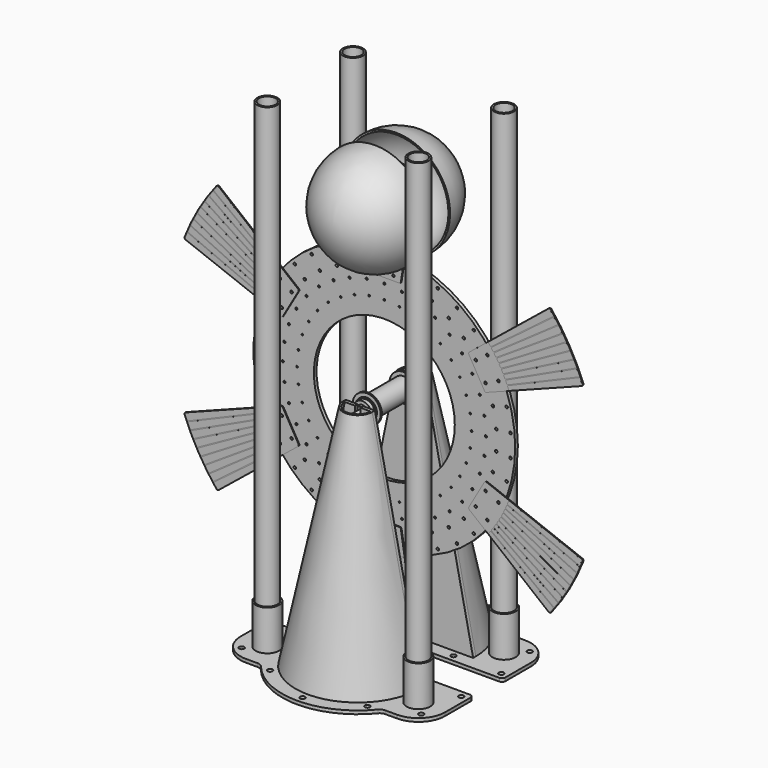
from build123d import *

# Parameters (mm, degrees)
F0_R      = 247.65
F0_R_2    = 2.38125
F0_R_3    = 1.9939
F0_R_4    = 1.5875
F0_R_5    = 133.35
F1_DEPTH  = 3.175
F2_R      = 2.38125
F3_DEPTH  = 1.5875
F5_DEPTH  = 0.0254
F8_COUNT  = 6
F13_DEPTH = 6.35
F14_DEPTH = 6.35
F15_ANGLE = 180
F16_R     = 4.7625
F16_R_2   = 22.225
F16_R_3   = 19.05
F16_R_4   = 15.875
F17_DEPTH = 6.35
F18_DEPTH = 76.2
F19_DEPTH = 908.05


with BuildPart() as f1:
    # F0 (on Front) → F1 (new body, symmetric)
    with BuildSketch(Plane.XZ):
        Circle(F0_R)
        with Locations((-137.4934414988, -196.3609844166)):
            Circle(F0_R_2, mode=Mode.SUBTRACT)
        with Locations((-196.3609844166, -137.4934414988)):
            Circle(F0_R_2, mode=Mode.SUBTRACT)
        with Locations((-169.5023342852, -169.5023342852)):
            Circle(F0_R_2, mode=Mode.SUBTRACT)
        with Locations((-150.4192900279, -150.4192900279)):
            Circle(F0_R_2, mode=Mode.SUBTRACT)
        with Locations((-101.3068800675, -217.2533054)):
            Circle(F0_R_2, mode=Mode.SUBTRACT)
        with Locations((-62.0421603491, -231.5444946343)):
            Circle(F0_R_2, mode=Mode.SUBTRACT)
        with Locations((-89.9014697288, -192.7943239974)):
            Circle(F0_R_2, mode=Mode.SUBTRACT)
        with Locations((-20.8923209834, -238.8003215663)):
            Circle(F0_R_2, mode=Mode.SUBTRACT)
        with Locations((-55.0572813694, -205.4765713973)):
            Circle(F0_R_2, mode=Mode.SUBTRACT)
        with Locations((-33.3715277272, -189.2593384922)):
            Circle(F0_R_3, mode=Mode.SUBTRACT)
        with Locations((-18.540205376, -211.9155171516)):
            Circle(F0_R_2, mode=Mode.SUBTRACT)
        with Locations((-122.0140474228, -174.2541186214)):
            Circle(F0_R_2, mode=Mode.SUBTRACT)
        with Locations((-96.0894844264, -166.4318690996)):
            Circle(F0_R_3, mode=Mode.SUBTRACT)
        with Locations((-65.7290784712, -180.5891589012)):
            Circle(F0_R_3, mode=Mode.SUBTRACT)
        with Locations((-123.5302600209, -147.217631174)):
            Circle(F0_R_3, mode=Mode.SUBTRACT)
        with Locations((-106.1242343592, -126.4739375589)):
            Circle(F0_R_4, mode=Mode.SUBTRACT)
        with Locations((-82.55, -142.9807941648)):
            Circle(F0_R_4, mode=Mode.SUBTRACT)
        with Locations((-56.4675256631, -155.1432516918)):
            Circle(F0_R_4, mode=Mode.SUBTRACT)
        with Locations((-28.6693141328, -162.5917600223)):
            Circle(F0_R_4, mode=Mode.SUBTRACT)
        with Locations((-217.2533054, -101.3068800675)):
            Circle(F0_R_2, mode=Mode.SUBTRACT)
        with Locations((-231.5444946343, -62.0421603491)):
            Circle(F0_R_2, mode=Mode.SUBTRACT)
        with Locations((-192.7943239974, -89.9014697288)):
            Circle(F0_R_2, mode=Mode.SUBTRACT)
        with Locations((-174.2541186214, -122.0140474228)):
            Circle(F0_R_2, mode=Mode.SUBTRACT)
        with Locations((-166.4318690996, -96.0894844264)):
            Circle(F0_R_3, mode=Mode.SUBTRACT)
        with Locations((-147.217631174, -123.5302600209)):
            Circle(F0_R_3, mode=Mode.SUBTRACT)
        with Locations((-126.4739375589, -106.1242343592)):
            Circle(F0_R_4, mode=Mode.SUBTRACT)
        with Locations((-180.5891589012, -65.7290784712)):
            Circle(F0_R_3, mode=Mode.SUBTRACT)
        with Locations((-142.9807941648, -82.55)):
            Circle(F0_R_4, mode=Mode.SUBTRACT)
        with Locations((-205.4765713973, -55.0572813694)):
            Circle(F0_R_2, mode=Mode.SUBTRACT)
        with Locations((-189.2593384922, -33.3715277272)):
            Circle(F0_R_3, mode=Mode.SUBTRACT)
        with Locations((-238.8003215663, -20.8923209834)):
            Circle(F0_R_2, mode=Mode.SUBTRACT)
        with Locations((-211.9155171516, -18.540205376)):
            Circle(F0_R_2, mode=Mode.SUBTRACT)
        with Locations((-155.1432516918, -56.4675256631)):
            Circle(F0_R_4, mode=Mode.SUBTRACT)
        with Locations((-162.5917600223, -28.6693141328)):
            Circle(F0_R_4, mode=Mode.SUBTRACT)
        with Locations((20.8923209834, -238.8003215663)):
            Circle(F0_R_2, mode=Mode.SUBTRACT)
        with Locations((18.540205376, -211.9155171516)):
            Circle(F0_R_2, mode=Mode.SUBTRACT)
        with Locations((0, -192.1789688528)):
            Circle(F0_R_3, mode=Mode.SUBTRACT)
        with Locations((55.0572813694, -205.4765713973)):
            Circle(F0_R_2, mode=Mode.SUBTRACT)
        with Locations((33.3715277272, -189.2593384922)):
            Circle(F0_R_3, mode=Mode.SUBTRACT)
        with Locations((62.0421603491, -231.5444946343)):
            Circle(F0_R_2, mode=Mode.SUBTRACT)
        with Locations((101.3068800675, -217.2533054)):
            Circle(F0_R_2, mode=Mode.SUBTRACT)
        with Locations((89.9014697288, -192.7943239974)):
            Circle(F0_R_2, mode=Mode.SUBTRACT)
        with Locations((0, -165.1)):
            Circle(F0_R_4, mode=Mode.SUBTRACT)
        with Locations((28.6693141328, -162.5917600223)):
            Circle(F0_R_4, mode=Mode.SUBTRACT)
        with Locations((56.4675256631, -155.1432516918)):
            Circle(F0_R_4, mode=Mode.SUBTRACT)
        with Locations((65.7290784712, -180.5891589012)):
            Circle(F0_R_3, mode=Mode.SUBTRACT)
        with Locations((122.0140474228, -174.2541186214)):
            Circle(F0_R_2, mode=Mode.SUBTRACT)
        with Locations((96.0894844264, -166.4318690996)):
            Circle(F0_R_3, mode=Mode.SUBTRACT)
        with Locations((82.55, -142.9807941648)):
            Circle(F0_R_4, mode=Mode.SUBTRACT)
        with Locations((123.5302600209, -147.217631174)):
            Circle(F0_R_3, mode=Mode.SUBTRACT)
        with Locations((106.1242343592, -126.4739375589)):
            Circle(F0_R_4, mode=Mode.SUBTRACT)
        with Locations((137.4934414988, -196.3609844166)):
            Circle(F0_R_2, mode=Mode.SUBTRACT)
        with Locations((169.5023342852, -169.5023342852)):
            Circle(F0_R_2, mode=Mode.SUBTRACT)
        with Locations((150.4192900279, -150.4192900279)):
            Circle(F0_R_2, mode=Mode.SUBTRACT)
        with Locations((196.3609844166, -137.4934414988)):
            Circle(F0_R_2, mode=Mode.SUBTRACT)
        with Locations((147.217631174, -123.5302600209)):
            Circle(F0_R_3, mode=Mode.SUBTRACT)
        with Locations((126.4739375589, -106.1242343592)):
            Circle(F0_R_4, mode=Mode.SUBTRACT)
        with Locations((174.2541186214, -122.0140474228)):
            Circle(F0_R_2, mode=Mode.SUBTRACT)
        with Locations((166.4318690996, -96.0894844264)):
            Circle(F0_R_3, mode=Mode.SUBTRACT)
        with Locations((142.9807941648, -82.55)):
            Circle(F0_R_4, mode=Mode.SUBTRACT)
        with Locations((180.5891589012, -65.7290784712)):
            Circle(F0_R_3, mode=Mode.SUBTRACT)
        with Locations((217.2533054, -101.3068800675)):
            Circle(F0_R_2, mode=Mode.SUBTRACT)
        with Locations((192.7943239974, -89.9014697288)):
            Circle(F0_R_2, mode=Mode.SUBTRACT)
        with Locations((231.5444946343, -62.0421603491)):
            Circle(F0_R_2, mode=Mode.SUBTRACT)
        with Locations((155.1432516918, -56.4675256631)):
            Circle(F0_R_4, mode=Mode.SUBTRACT)
        with Locations((162.5917600223, -28.6693141328)):
            Circle(F0_R_4, mode=Mode.SUBTRACT)
        with Locations((205.4765713973, -55.0572813694)):
            Circle(F0_R_2, mode=Mode.SUBTRACT)
        with Locations((189.2593384922, -33.3715277272)):
            Circle(F0_R_3, mode=Mode.SUBTRACT)
        with Locations((211.9155171516, -18.540205376)):
            Circle(F0_R_2, mode=Mode.SUBTRACT)
        with Locations((238.8003215663, -20.8923209834)):
            Circle(F0_R_2, mode=Mode.SUBTRACT)
        with Locations((-238.8003215663, 20.8923209834)):
            Circle(F0_R_2, mode=Mode.SUBTRACT)
        with Locations((-192.1789688528, 0)):
            Circle(F0_R_3, mode=Mode.SUBTRACT)
        with Locations((-211.9155171516, 18.540205376)):
            Circle(F0_R_2, mode=Mode.SUBTRACT)
        with Locations((-189.2593384922, 33.3715277272)):
            Circle(F0_R_3, mode=Mode.SUBTRACT)
        with Locations((-205.4765713973, 55.0572813694)):
            Circle(F0_R_2, mode=Mode.SUBTRACT)
        with Locations((-165.1, 0)):
            Circle(F0_R_4, mode=Mode.SUBTRACT)
        with Locations((-162.5917600223, 28.6693141328)):
            Circle(F0_R_4, mode=Mode.SUBTRACT)
        with Locations((-155.1432516918, 56.4675256631)):
            Circle(F0_R_4, mode=Mode.SUBTRACT)
        with Locations((-231.5444946343, 62.0421603491)):
            Circle(F0_R_2, mode=Mode.SUBTRACT)
        with Locations((-192.7943239974, 89.9014697288)):
            Circle(F0_R_2, mode=Mode.SUBTRACT)
        with Locations((-217.2533054, 101.3068800675)):
            Circle(F0_R_2, mode=Mode.SUBTRACT)
        with Locations((-180.5891589012, 65.7290784712)):
            Circle(F0_R_3, mode=Mode.SUBTRACT)
        with Locations((-142.9807941648, 82.55)):
            Circle(F0_R_4, mode=Mode.SUBTRACT)
        with Locations((-166.4318690996, 96.0894844264)):
            Circle(F0_R_3, mode=Mode.SUBTRACT)
        with Locations((-174.2541186214, 122.0140474228)):
            Circle(F0_R_2, mode=Mode.SUBTRACT)
        with Locations((-126.4739375589, 106.1242343592)):
            Circle(F0_R_4, mode=Mode.SUBTRACT)
        with Locations((-147.217631174, 123.5302600209)):
            Circle(F0_R_3, mode=Mode.SUBTRACT)
        with Locations((-196.3609844166, 137.4934414988)):
            Circle(F0_R_2, mode=Mode.SUBTRACT)
        with Locations((-150.4192900279, 150.4192900279)):
            Circle(F0_R_2, mode=Mode.SUBTRACT)
        with Locations((-169.5023342852, 169.5023342852)):
            Circle(F0_R_2, mode=Mode.SUBTRACT)
        with Locations((-137.4934414988, 196.3609844166)):
            Circle(F0_R_2, mode=Mode.SUBTRACT)
        with Locations((-106.1242343592, 126.4739375589)):
            Circle(F0_R_4, mode=Mode.SUBTRACT)
        with Locations((-123.5302600209, 147.217631174)):
            Circle(F0_R_3, mode=Mode.SUBTRACT)
        with Locations((-82.55, 142.9807941648)):
            Circle(F0_R_4, mode=Mode.SUBTRACT)
        with Locations((-96.0894844264, 166.4318690996)):
            Circle(F0_R_3, mode=Mode.SUBTRACT)
        with Locations((-122.0140474228, 174.2541186214)):
            Circle(F0_R_2, mode=Mode.SUBTRACT)
        with Locations((-65.7290784712, 180.5891589012)):
            Circle(F0_R_3, mode=Mode.SUBTRACT)
        with Locations((-56.4675256631, 155.1432516918)):
            Circle(F0_R_4, mode=Mode.SUBTRACT)
        with Locations((-28.6693141328, 162.5917600223)):
            Circle(F0_R_4, mode=Mode.SUBTRACT)
        with Locations((-89.9014697288, 192.7943239974)):
            Circle(F0_R_2, mode=Mode.SUBTRACT)
        with Locations((-101.3068800675, 217.2533054)):
            Circle(F0_R_2, mode=Mode.SUBTRACT)
        with Locations((-62.0421603491, 231.5444946343)):
            Circle(F0_R_2, mode=Mode.SUBTRACT)
        with Locations((-33.3715277272, 189.2593384922)):
            Circle(F0_R_3, mode=Mode.SUBTRACT)
        with Locations((-55.0572813694, 205.4765713973)):
            Circle(F0_R_2, mode=Mode.SUBTRACT)
        with Locations((-18.540205376, 211.9155171516)):
            Circle(F0_R_2, mode=Mode.SUBTRACT)
        with Locations((-20.8923209834, 238.8003215663)):
            Circle(F0_R_2, mode=Mode.SUBTRACT)
        Circle(F0_R_5, mode=Mode.SUBTRACT)
        with Locations((165.1, 0)):
            Circle(F0_R_4, mode=Mode.SUBTRACT)
        with Locations((162.5917600223, 28.6693141328)):
            Circle(F0_R_4, mode=Mode.SUBTRACT)
        with Locations((155.1432516918, 56.4675256631)):
            Circle(F0_R_4, mode=Mode.SUBTRACT)
        with Locations((192.1789688528, 0)):
            Circle(F0_R_3, mode=Mode.SUBTRACT)
        with Locations((211.9155171516, 18.540205376)):
            Circle(F0_R_2, mode=Mode.SUBTRACT)
        with Locations((238.8003215663, 20.8923209834)):
            Circle(F0_R_2, mode=Mode.SUBTRACT)
        with Locations((189.2593384922, 33.3715277272)):
            Circle(F0_R_3, mode=Mode.SUBTRACT)
        with Locations((205.4765713973, 55.0572813694)):
            Circle(F0_R_2, mode=Mode.SUBTRACT)
        with Locations((142.9807941648, 82.55)):
            Circle(F0_R_4, mode=Mode.SUBTRACT)
        with Locations((180.5891589012, 65.7290784712)):
            Circle(F0_R_3, mode=Mode.SUBTRACT)
        with Locations((126.4739375589, 106.1242343592)):
            Circle(F0_R_4, mode=Mode.SUBTRACT)
        with Locations((147.217631174, 123.5302600209)):
            Circle(F0_R_3, mode=Mode.SUBTRACT)
        with Locations((166.4318690996, 96.0894844264)):
            Circle(F0_R_3, mode=Mode.SUBTRACT)
        with Locations((174.2541186214, 122.0140474228)):
            Circle(F0_R_2, mode=Mode.SUBTRACT)
        with Locations((192.7943239974, 89.9014697288)):
            Circle(F0_R_2, mode=Mode.SUBTRACT)
        with Locations((231.5444946343, 62.0421603491)):
            Circle(F0_R_2, mode=Mode.SUBTRACT)
        with Locations((217.2533054, 101.3068800675)):
            Circle(F0_R_2, mode=Mode.SUBTRACT)
        with Locations((0, 165.1)):
            Circle(F0_R_4, mode=Mode.SUBTRACT)
        with Locations((28.6693141328, 162.5917600223)):
            Circle(F0_R_4, mode=Mode.SUBTRACT)
        with Locations((56.4675256631, 155.1432516918)):
            Circle(F0_R_4, mode=Mode.SUBTRACT)
        with Locations((82.55, 142.9807941648)):
            Circle(F0_R_4, mode=Mode.SUBTRACT)
        with Locations((106.1242343592, 126.4739375589)):
            Circle(F0_R_4, mode=Mode.SUBTRACT)
        with Locations((123.5302600209, 147.217631174)):
            Circle(F0_R_3, mode=Mode.SUBTRACT)
        with Locations((65.7290784712, 180.5891589012)):
            Circle(F0_R_3, mode=Mode.SUBTRACT)
        with Locations((96.0894844264, 166.4318690996)):
            Circle(F0_R_3, mode=Mode.SUBTRACT)
        with Locations((122.0140474228, 174.2541186214)):
            Circle(F0_R_2, mode=Mode.SUBTRACT)
        with Locations((0, 192.1789688528)):
            Circle(F0_R_3, mode=Mode.SUBTRACT)
        with Locations((18.540205376, 211.9155171516)):
            Circle(F0_R_2, mode=Mode.SUBTRACT)
        with Locations((33.3715277272, 189.2593384922)):
            Circle(F0_R_3, mode=Mode.SUBTRACT)
        with Locations((55.0572813694, 205.4765713973)):
            Circle(F0_R_2, mode=Mode.SUBTRACT)
        with Locations((20.8923209834, 238.8003215663)):
            Circle(F0_R_2, mode=Mode.SUBTRACT)
        with Locations((89.9014697288, 192.7943239974)):
            Circle(F0_R_2, mode=Mode.SUBTRACT)
        with Locations((62.0421603491, 231.5444946343)):
            Circle(F0_R_2, mode=Mode.SUBTRACT)
        with Locations((101.3068800675, 217.2533054)):
            Circle(F0_R_2, mode=Mode.SUBTRACT)
        with Locations((150.4192900279, 150.4192900279)):
            Circle(F0_R_2, mode=Mode.SUBTRACT)
        with Locations((169.5023342852, 169.5023342852)):
            Circle(F0_R_2, mode=Mode.SUBTRACT)
        with Locations((196.3609844166, 137.4934414988)):
            Circle(F0_R_2, mode=Mode.SUBTRACT)
        with Locations((137.4934414988, 196.3609844166)):
            Circle(F0_R_2, mode=Mode.SUBTRACT)
    extrude(amount=F1_DEPTH, both=True)


with BuildPart() as f3:
    # F2 (on face) → F3 (new body)
    with BuildSketch(Plane.XZ.offset(3.175)):
        with BuildLine():
            ThreePointArc((-60.1639478818, 400.3166990416), (-62.2533062589, 399.0533165864), (-62.8279842621, 396.680280799))
            Line((-62.8279842621, 396.680280799), (-38.7409952672, 244.6010175484))
            ThreePointArc((-38.7409952672, 244.6010175484), (0, 247.65), (38.7409952672, 244.6010175484))
            Line((38.7409952672, 244.6010175484), (62.8279842621, 396.680280799))
            ThreePointArc((62.8279842621, 396.680280799), (62.2533062589, 399.0533165864), (60.1639478818, 400.3166990416))
            ThreePointArc((60.1639478818, 400.3166990416), (0, 404.8125), (-60.1639478818, 400.3166990416))
        make_face()
        with BuildLine():
            ThreePointArc((38.7409952672, 244.6010175484), (0, 247.65), (-38.7409952672, 244.6010175484))
            Line((-38.7409952672, 244.6010175484), (-32.607922579, 205.8783205735))
            ThreePointArc((-32.607922579, 205.8783205735), (-31.534009651, 203.9607110592), (-29.4720120976, 203.2))
            Line((-29.4720120976, 203.2), (29.4720120976, 203.2))
            ThreePointArc((29.4720120976, 203.2), (31.534009651, 203.9607110592), (32.607922579, 205.8783205735))
            Line((32.607922579, 205.8783205735), (38.7409952672, 244.6010175484))
        make_face()
        with Locations((-18.540205376, 211.9155171516)):
            Circle(F2_R, mode=Mode.SUBTRACT)
        with Locations((-20.8923209834, 238.8003215663)):
            Circle(F2_R, mode=Mode.SUBTRACT)
        with Locations((18.540205376, 211.9155171516)):
            Circle(F2_R, mode=Mode.SUBTRACT)
        with Locations((20.8923209834, 238.8003215663)):
            Circle(F2_R, mode=Mode.SUBTRACT)
    extrude(amount=F3_DEPTH)


with BuildPart() as f5:
    # F4 (on face) → F5 (new body)
    with BuildSketch(Plane.XZ.offset(4.7625)):
        with BuildLine():
            ThreePointArc((-60.4953058214, 398.6469171423), (-61.5378093397, 398.0144293509), (-61.8242218909, 396.8291773766))
            Line((-61.8242218909, 396.8291773766), (-38.9763372282, 252.5733109802))
            ThreePointArc((-38.9763372282, 252.5733109802), (-38.3474638471, 251.541696979), (-37.1746613313, 251.2514497812))
            ThreePointArc((-37.1746613313, 251.2514497812), (-35.1293239896, 251.5473932788), (-33.0816464646, 251.826685507))
            ThreePointArc((-33.0816464646, 251.826685507), (-32.0342792994, 252.428957205), (-31.7141187621, 253.5939492252))
            Line((-31.7141187621, 253.5939492252), (-49.5136279772, 398.5593185209))
            ThreePointArc((-49.5136279772, 398.5593185209), (-50.115645112, 399.6197098456), (-51.2921010745, 399.9403432193))
            ThreePointArc((-51.2921010745, 399.9403432193), (-55.8974299804, 399.3201458367), (-60.4953058214, 398.6469171423))
        make_face()
    extrude(amount=F5_DEPTH)


with BuildPart() as f5b:
    # F4 (on face) → F5, piece 2 (new body)
    with BuildSketch(Plane.XZ.offset(4.7625)):
        with BuildLine():
            ThreePointArc((-46.6012907559, 400.5153279375), (-47.6652327148, 399.9196082886), (-47.9928354886, 398.7450739917))
            Line((-47.9928354886, 398.7450739917), (-30.1933262735, 253.779704696))
            ThreePointArc((-30.1933262735, 253.779704696), (-29.6008387945, 252.7267717617), (-28.4388801995, 252.3957711571))
            ThreePointArc((-28.4388801995, 252.3957711571), (-26.3844605429, 252.6201531301), (-24.3282832495, 252.827812306))
            ThreePointArc((-24.3282832495, 252.827812306), (-23.260535133, 253.3931645294), (-22.8999119936, 254.5462734264))
            Line((-22.8999119936, 254.5462734264), (-35.6293598009, 400.0445276491))
            ThreePointArc((-35.6293598009, 400.0445276491), (-36.1940030796, 401.125283107), (-37.3585524336, 401.4867788806))
            ThreePointArc((-37.3585524336, 401.4867788806), (-41.982720474, 401.0276829665), (-46.6012907559, 400.5153279375))
        make_face()
    extrude(amount=F5_DEPTH)


with BuildPart() as f5c:
    # F4 (on face) → F5, piece 3 (new body)
    with BuildSketch(Plane.XZ.offset(4.7625)):
        with BuildLine():
            ThreePointArc((-32.6505329525, 401.8977064143), (-33.7346171027, 401.3394807007), (-34.1030109656, 400.1770950702))
            Line((-34.1030109656, 400.1770950702), (-21.3735631583, 254.6788408475))
            ThreePointArc((-21.3735631583, 254.6788408475), (-20.8181834361, 253.6058718167), (-19.6684844294, 253.2345210785))
            ThreePointArc((-19.6684844294, 253.2345210785), (-17.6074854518, 253.3870681521), (-15.5453135253, 253.522841275))
            ThreePointArc((-15.5453135253, 253.522841275), (-14.458485344, 254.0505852292), (-14.0578389664, 255.1904061173))
            Line((-14.0578389664, 255.1904061173), (-21.7017164946, 401.0442780566))
            ThreePointArc((-21.7017164946, 401.0442780566), (-22.2282979863, 402.1440809137), (-23.3795219077, 402.5459986602))
            ThreePointArc((-23.3795219077, 402.5459986602), (-28.0168952462, 402.2485635521), (-32.6505329525, 401.8977064143))
        make_face()
    extrude(amount=F5_DEPTH)


with BuildPart() as f5d:
    # F4 (on face) → F5, piece 4 (new body)
    with BuildSketch(Plane.XZ.offset(4.7625)):
        with BuildLine():
            ThreePointArc((-18.6600292608, 402.7923683576), (-19.7629348127, 402.2723166912), (-20.1716709334, 401.1234959151))
            Line((-20.1716709334, 401.1234959151), (-12.5277934053, 255.2696239758))
            ThreePointArc((-12.5277934053, 255.2696239758), (-12.0101980846, 254.177926096), (-10.8741593973, 253.766677658))
            ThreePointArc((-10.8741593973, 253.766677658), (-8.8090921085, 253.8472039769), (-6.7434379878, 253.9109256281))
            ThreePointArc((-6.7434379878, 253.9109256281), (-5.6388538745, 254.4004183385), (-5.1986723845, 255.5255625216))
            Line((-5.1986723845, 255.5255625216), (-7.7476667462, 401.5573517015))
            ThreePointArc((-7.7476667462, 401.5573517015), (-8.2355448926, 402.6748620175), (-9.3720407924, 403.1167120619))
            ThreePointArc((-9.3720407924, 403.1167120619), (-14.0169695039, 402.9813001389), (-18.6600292608, 402.7923683576))
        make_face()
    extrude(amount=F5_DEPTH)


with BuildPart() as f5e:
    # F4 (on face) → F5, piece 5 (new body)
    with BuildSketch(Plane.XZ.offset(4.7625)):
        with BuildLine():
            ThreePointArc((-4.6468249545, 403.1982237595), (-5.7672081875, 402.7169797433), (-6.2157885841, 401.5831234826))
            Line((-6.2157885841, 401.5831234826), (-3.6667942224, 255.5513343027))
            ThreePointArc((-3.6667942224, 255.5513343027), (-3.1876139133, 254.4422376395), (-2.0666196336, 253.9915925445))
            ThreePointArc((-2.0666196336, 253.9915925445), (0, 254), (2.0666196336, 253.9915925445))
            ThreePointArc((2.0666196336, 253.9915925445), (3.1876139133, 254.4422376395), (3.6667942224, 255.5513343027))
            Line((3.6667942224, 255.5513343027), (6.2157885841, 401.5831234826))
            ThreePointArc((6.2157885841, 401.5831234826), (5.7672081875, 402.7169797433), (4.6468249545, 403.1982237595))
            ThreePointArc((4.6468249545, 403.1982237595), (0, 403.225), (-4.6468249545, 403.1982237595))
        make_face()
    extrude(amount=F5_DEPTH)


with BuildPart() as f5f:
    # F4 (on face) → F5, piece 6 (new body)
    with BuildSketch(Plane.XZ.offset(4.7625)):
        with BuildLine():
            ThreePointArc((9.4274208463, 403.1147781478), (8.2909249465, 402.6729281034), (7.8030468001, 401.5554177874))
            Line((7.8030468001, 401.5554177874), (5.2540524384, 255.5236286075))
            ThreePointArc((5.2540524384, 255.5236286075), (5.6942339284, 254.3984844244), (6.7988180417, 253.908991714))
            ThreePointArc((6.7988180417, 253.908991714), (8.8644721624, 253.8452700629), (10.9295394512, 253.7647437439))
            ThreePointArc((10.9295394512, 253.7647437439), (12.0655781385, 254.1759921819), (12.5831734592, 255.2676900617))
            Line((12.5831734592, 255.2676900617), (20.2270509874, 401.121562001))
            ThreePointArc((20.2270509874, 401.121562001), (19.8183148667, 402.2703827771), (18.7154093148, 402.7904344435))
            ThreePointArc((18.7154093148, 402.7904344435), (14.0723495579, 402.9793662248), (9.4274208463, 403.1147781478))
        make_face()
    extrude(amount=F5_DEPTH)


with BuildPart() as f5g:
    # F4 (on face) → F5, piece 7 (new body)
    with BuildSketch(Plane.XZ.offset(4.7625)):
        with BuildLine():
            ThreePointArc((23.4901807869, 402.5401992741), (22.3389568656, 402.1382815276), (21.8123753738, 401.0384786704))
            Line((21.8123753738, 401.0384786704), (14.1684978456, 255.1846067312))
            ThreePointArc((14.1684978456, 255.1846067312), (14.5691442233, 254.0447858431), (15.6559724045, 253.5170418888))
            ThreePointArc((15.6559724045, 253.5170418888), (17.718144331, 253.381268766), (19.7791433086, 253.2287216924))
            ThreePointArc((19.7791433086, 253.2287216924), (20.9288423153, 253.6000724306), (21.4842220375, 254.6730414614))
            Line((21.4842220375, 254.6730414614), (34.2136698448, 400.1712956841))
            ThreePointArc((34.2136698448, 400.1712956841), (33.845275982, 401.3336813146), (32.7611918318, 401.8919070282))
            ThreePointArc((32.7611918318, 401.8919070282), (28.1275541255, 402.242764166), (23.4901807869, 402.5401992741))
        make_face()
    extrude(amount=F5_DEPTH)


with BuildPart() as f5h:
    # F4 (on face) → F5, piece 8 (new body)
    with BuildSketch(Plane.XZ.offset(4.7625)):
        with BuildLine():
            ThreePointArc((37.5243215607, 401.475187174), (36.3597722067, 401.1136914004), (35.795128928, 400.0329359425))
            Line((35.795128928, 400.0329359425), (23.0656811207, 254.5346817198))
            ThreePointArc((23.0656811207, 254.5346817198), (23.4263042601, 253.3815728229), (24.4940523766, 252.8162205994))
            ThreePointArc((24.4940523766, 252.8162205994), (26.55022967, 252.6085614235), (28.6046493266, 252.3841794505))
            ThreePointArc((28.6046493266, 252.3841794505), (29.7666079216, 252.7151800552), (30.3590954006, 253.7681129894))
            Line((30.3590954006, 253.7681129894), (48.1586046157, 398.7334822851))
            ThreePointArc((48.1586046157, 398.7334822851), (47.831001842, 399.9080165821), (46.767059883, 400.5037362309))
            ThreePointArc((46.767059883, 400.5037362309), (42.1484896011, 401.0160912599), (37.5243215607, 401.475187174))
        make_face()
    extrude(amount=F5_DEPTH)


with BuildPart() as f5i:
    # F4 (on face) → F5, piece 9 (new body)
    with BuildSketch(Plane.XZ.offset(4.7625)):
        with BuildLine():
            ThreePointArc((51.5127447288, 399.9210394009), (50.3362887663, 399.6004060271), (49.7342716314, 398.5400147025))
            Line((49.7342716314, 398.5400147025), (31.9347624163, 253.5746454068))
            ThreePointArc((31.9347624163, 253.5746454068), (32.2549229537, 252.4096533866), (33.3022901188, 251.8073816885))
            ThreePointArc((33.3022901188, 251.8073816885), (35.3499676439, 251.5280894604), (37.3953049856, 251.2321459627))
            ThreePointArc((37.3953049856, 251.2321459627), (38.5681075013, 251.5223931606), (39.1969808824, 252.5540071617))
            Line((39.1969808824, 252.5540071617), (62.0448655452, 396.8098735581))
            ThreePointArc((62.0448655452, 396.8098735581), (61.758452994, 397.9951255325), (60.7159494756, 398.6276133239))
            ThreePointArc((60.7159494756, 398.6276133239), (56.1180736346, 399.3008420183), (51.5127447288, 399.9210394009))
        make_face()
    extrude(amount=F5_DEPTH)


with BuildPart() as f7:
    # F6 (on Right) → F7 (revolve)
    with BuildSketch(Plane.YZ):
        with BuildLine():
            Line((-25.4, 428.625), (-25.4, 431.8))
            ThreePointArc((-25.4, 431.8), (-97.2420489686, 402.0420489686), (-127, 330.2))
            Line((-127, 330.2), (-123.825, 330.2))
            ThreePointArc((-123.825, 330.2), (-94.9969849383, 399.7969849383), (-25.4, 428.625))
        make_face()
    revolve(axis=Axis((0, -125.4125, 330.2), (0, 1, 0)))


with BuildPart() as f8_1:
    # F8: instance of F5
    add(f5.part.rotate(Axis((0, 3.175, 0), (0, -1, 0)), 1 * 360 / F8_COUNT))


with BuildPart() as f8_2:
    # F8: instance of F5
    add(f5.part.rotate(Axis((0, 3.175, 0), (0, -1, 0)), 2 * 360 / F8_COUNT))


with BuildPart() as f8_3:
    # F8: instance of F5
    add(f5.part.rotate(Axis((0, 3.175, 0), (0, -1, 0)), 3 * 360 / F8_COUNT))


with BuildPart() as f8_4:
    # F8: instance of F5
    add(f5.part.rotate(Axis((0, 3.175, 0), (0, -1, 0)), 4 * 360 / F8_COUNT))


with BuildPart() as f8_5:
    # F8: instance of F5
    add(f5.part.rotate(Axis((0, 3.175, 0), (0, -1, 0)), 5 * 360 / F8_COUNT))


with BuildPart() as f8_6:
    # F8: instance of F5b
    add(f5b.part.rotate(Axis((0, 3.175, 0), (0, -1, 0)), 1 * 360 / F8_COUNT))


with BuildPart() as f8_7:
    # F8: instance of F5b
    add(f5b.part.rotate(Axis((0, 3.175, 0), (0, -1, 0)), 2 * 360 / F8_COUNT))


with BuildPart() as f8_8:
    # F8: instance of F5b
    add(f5b.part.rotate(Axis((0, 3.175, 0), (0, -1, 0)), 3 * 360 / F8_COUNT))


with BuildPart() as f8_9:
    # F8: instance of F5b
    add(f5b.part.rotate(Axis((0, 3.175, 0), (0, -1, 0)), 4 * 360 / F8_COUNT))


with BuildPart() as f8_10:
    # F8: instance of F5b
    add(f5b.part.rotate(Axis((0, 3.175, 0), (0, -1, 0)), 5 * 360 / F8_COUNT))


with BuildPart() as f8_11:
    # F8: instance of F5c
    add(f5c.part.rotate(Axis((0, 3.175, 0), (0, -1, 0)), 1 * 360 / F8_COUNT))


with BuildPart() as f8_12:
    # F8: instance of F5c
    add(f5c.part.rotate(Axis((0, 3.175, 0), (0, -1, 0)), 2 * 360 / F8_COUNT))


with BuildPart() as f8_13:
    # F8: instance of F5c
    add(f5c.part.rotate(Axis((0, 3.175, 0), (0, -1, 0)), 3 * 360 / F8_COUNT))


with BuildPart() as f8_14:
    # F8: instance of F5c
    add(f5c.part.rotate(Axis((0, 3.175, 0), (0, -1, 0)), 4 * 360 / F8_COUNT))


with BuildPart() as f8_15:
    # F8: instance of F5c
    add(f5c.part.rotate(Axis((0, 3.175, 0), (0, -1, 0)), 5 * 360 / F8_COUNT))


with BuildPart() as f8_16:
    # F8: instance of F5d
    add(f5d.part.rotate(Axis((0, 3.175, 0), (0, -1, 0)), 1 * 360 / F8_COUNT))


with BuildPart() as f8_17:
    # F8: instance of F5d
    add(f5d.part.rotate(Axis((0, 3.175, 0), (0, -1, 0)), 2 * 360 / F8_COUNT))


with BuildPart() as f8_18:
    # F8: instance of F5d
    add(f5d.part.rotate(Axis((0, 3.175, 0), (0, -1, 0)), 3 * 360 / F8_COUNT))


with BuildPart() as f8_19:
    # F8: instance of F5d
    add(f5d.part.rotate(Axis((0, 3.175, 0), (0, -1, 0)), 4 * 360 / F8_COUNT))


with BuildPart() as f8_20:
    # F8: instance of F5d
    add(f5d.part.rotate(Axis((0, 3.175, 0), (0, -1, 0)), 5 * 360 / F8_COUNT))


with BuildPart() as f8_21:
    # F8: instance of F5i
    add(f5i.part.rotate(Axis((0, 3.175, 0), (0, -1, 0)), 1 * 360 / F8_COUNT))


with BuildPart() as f8_22:
    # F8: instance of F5i
    add(f5i.part.rotate(Axis((0, 3.175, 0), (0, -1, 0)), 2 * 360 / F8_COUNT))


with BuildPart() as f8_23:
    # F8: instance of F5i
    add(f5i.part.rotate(Axis((0, 3.175, 0), (0, -1, 0)), 3 * 360 / F8_COUNT))


with BuildPart() as f8_24:
    # F8: instance of F5i
    add(f5i.part.rotate(Axis((0, 3.175, 0), (0, -1, 0)), 4 * 360 / F8_COUNT))


with BuildPart() as f8_25:
    # F8: instance of F5i
    add(f5i.part.rotate(Axis((0, 3.175, 0), (0, -1, 0)), 5 * 360 / F8_COUNT))


with BuildPart() as f8_26:
    # F8: instance of F5h
    add(f5h.part.rotate(Axis((0, 3.175, 0), (0, -1, 0)), 1 * 360 / F8_COUNT))


with BuildPart() as f8_27:
    # F8: instance of F5h
    add(f5h.part.rotate(Axis((0, 3.175, 0), (0, -1, 0)), 2 * 360 / F8_COUNT))


with BuildPart() as f8_28:
    # F8: instance of F5h
    add(f5h.part.rotate(Axis((0, 3.175, 0), (0, -1, 0)), 3 * 360 / F8_COUNT))


with BuildPart() as f8_29:
    # F8: instance of F5h
    add(f5h.part.rotate(Axis((0, 3.175, 0), (0, -1, 0)), 4 * 360 / F8_COUNT))


with BuildPart() as f8_30:
    # F8: instance of F5h
    add(f5h.part.rotate(Axis((0, 3.175, 0), (0, -1, 0)), 5 * 360 / F8_COUNT))


with BuildPart() as f8_31:
    # F8: instance of F5g
    add(f5g.part.rotate(Axis((0, 3.175, 0), (0, -1, 0)), 1 * 360 / F8_COUNT))


with BuildPart() as f8_32:
    # F8: instance of F5g
    add(f5g.part.rotate(Axis((0, 3.175, 0), (0, -1, 0)), 2 * 360 / F8_COUNT))


with BuildPart() as f8_33:
    # F8: instance of F5g
    add(f5g.part.rotate(Axis((0, 3.175, 0), (0, -1, 0)), 3 * 360 / F8_COUNT))


with BuildPart() as f8_34:
    # F8: instance of F5g
    add(f5g.part.rotate(Axis((0, 3.175, 0), (0, -1, 0)), 4 * 360 / F8_COUNT))


with BuildPart() as f8_35:
    # F8: instance of F5g
    add(f5g.part.rotate(Axis((0, 3.175, 0), (0, -1, 0)), 5 * 360 / F8_COUNT))


with BuildPart() as f8_36:
    # F8: instance of F5e
    add(f5e.part.rotate(Axis((0, 3.175, 0), (0, -1, 0)), 1 * 360 / F8_COUNT))


with BuildPart() as f8_37:
    # F8: instance of F5e
    add(f5e.part.rotate(Axis((0, 3.175, 0), (0, -1, 0)), 2 * 360 / F8_COUNT))


with BuildPart() as f8_38:
    # F8: instance of F5e
    add(f5e.part.rotate(Axis((0, 3.175, 0), (0, -1, 0)), 3 * 360 / F8_COUNT))


with BuildPart() as f8_39:
    # F8: instance of F5e
    add(f5e.part.rotate(Axis((0, 3.175, 0), (0, -1, 0)), 4 * 360 / F8_COUNT))


with BuildPart() as f8_40:
    # F8: instance of F5e
    add(f5e.part.rotate(Axis((0, 3.175, 0), (0, -1, 0)), 5 * 360 / F8_COUNT))


with BuildPart() as f8_41:
    # F8: instance of F3
    add(f3.part.rotate(Axis((0, 3.175, 0), (0, -1, 0)), 1 * 360 / F8_COUNT))


with BuildPart() as f8_42:
    # F8: instance of F3
    add(f3.part.rotate(Axis((0, 3.175, 0), (0, -1, 0)), 2 * 360 / F8_COUNT))


with BuildPart() as f8_43:
    # F8: instance of F3
    add(f3.part.rotate(Axis((0, 3.175, 0), (0, -1, 0)), 3 * 360 / F8_COUNT))


with BuildPart() as f8_44:
    # F8: instance of F3
    add(f3.part.rotate(Axis((0, 3.175, 0), (0, -1, 0)), 4 * 360 / F8_COUNT))


with BuildPart() as f8_45:
    # F8: instance of F3
    add(f3.part.rotate(Axis((0, 3.175, 0), (0, -1, 0)), 5 * 360 / F8_COUNT))


with BuildPart() as f8_46:
    # F8: instance of F5f
    add(f5f.part.rotate(Axis((0, 3.175, 0), (0, -1, 0)), 1 * 360 / F8_COUNT))


with BuildPart() as f8_47:
    # F8: instance of F5f
    add(f5f.part.rotate(Axis((0, 3.175, 0), (0, -1, 0)), 2 * 360 / F8_COUNT))


with BuildPart() as f8_48:
    # F8: instance of F5f
    add(f5f.part.rotate(Axis((0, 3.175, 0), (0, -1, 0)), 3 * 360 / F8_COUNT))


with BuildPart() as f8_49:
    # F8: instance of F5f
    add(f5f.part.rotate(Axis((0, 3.175, 0), (0, -1, 0)), 4 * 360 / F8_COUNT))


with BuildPart() as f8_50:
    # F8: instance of F5f
    add(f5f.part.rotate(Axis((0, 3.175, 0), (0, -1, 0)), 5 * 360 / F8_COUNT))


with BuildPart() as f10:
    # F9 (on Top) → F10 (revolve)
    with BuildSketch(Plane.XY):
        Polygon((5, 80), (0, 80), (0, -80), (5, -80), (5, -60), (10, -60), (10, 60), (5, 60), align=None)
    revolve(axis=Axis((0, 0, 0), (0, 1, 0)))

    # F12 (on offset) → F13 (join)
    with BuildSketch(Plane.XZ.offset(66.35)):
        with BuildLine():
            ThreePointArc((5.25, 0), (0, -5.25), (-5.25, 0))
            Line((-5.25, 0), (-5.25, 12.7))
            Line((-5.25, 12.7), (-24.3, 12.7))
            Line((-24.3, 12.7), (-114.3, -419.1))
            Line((-114.3, -419.1), (114.3, -419.1))
            Line((114.3, -419.1), (24.3, 12.7))
            Line((24.3, 12.7), (5.25, 12.7))
            Line((5.25, 12.7), (5.25, 0))
        make_face()
    extrude(amount=-F13_DEPTH)

    # F12 (on offset) → F14 (join)
    with BuildSketch(Plane.XZ.offset(66.35)):
        Polygon((27.5432325735, 12.7), (24.3, 12.7), (114.3, -419.1), (117.5432325735, -419.1), align=None)
        Polygon((-114.3, -419.1), (-24.3, 12.7), (-27.5432325735, 12.7), (-117.5432325735, -419.1), align=None)
    extrude(amount=-F14_DEPTH)

    # F12 (on offset) → F15 (revolve)
    with BuildSketch(Plane.XZ.offset(66.35)):
        Polygon((27.5432325735, 12.7), (24.3, 12.7), (114.3, -419.1), (117.5432325735, -419.1), align=None)
    revolve(axis=Axis((0, -66.35, -209.55), (0, 0, -1)), revolution_arc=F15_ANGLE)

    # F16 (on face) → F17 (join)
    with BuildSketch(Plane(origin=(0, 0, -419.1), x_dir=(1, 0, 0), z_dir=(0, 0, -1))):
        with BuildLine():
            ThreePointArc((110.7326668834, 156.743828459), (61.2845073977, 195.4893700294), (0, 209.2932325735))
            ThreePointArc((0, 209.2932325735), (-61.2845073977, 195.4893700294), (-110.7326668834, 156.743828459))
            ThreePointArc((-110.7326668834, 156.743828459), (-115.1259607397, 153.3014243025), (-120.5708721912, 152.075))
            Line((-120.5708721912, 152.075), (-142.9432325735, 152.075))
            ThreePointArc((-142.9432325735, 152.075), (-178.8642570578, 137.1960244843), (-193.7432325735, 101.275))
            Line((-193.7432325735, 101.275), (-193.7432325735, 40.95))
            ThreePointArc((-193.7432325735, 40.95), (-191.8833606341, 36.4598719395), (-187.3932325735, 34.6))
            Line((-187.3932325735, 34.6), (0, 34.6))
            Line((0, 34.6), (187.3932325735, 34.6))
            ThreePointArc((187.3932325735, 34.6), (191.8833606341, 36.4598719395), (193.7432325735, 40.95))
            Line((193.7432325735, 40.95), (193.7432325735, 101.275))
            ThreePointArc((193.7432325735, 101.275), (178.8642570578, 137.1960244843), (142.9432325735, 152.075))
            Line((142.9432325735, 152.075), (120.5708721912, 152.075))
            ThreePointArc((120.5708721912, 152.075), (115.1259607397, 153.3014243025), (110.7326668834, 156.743828459))
        make_face()
        with Locations((-181.0432325735, 47.3)):
            Circle(F16_R, mode=Mode.SUBTRACT)
        with Locations((-90.5216162868, 47.3)):
            Circle(F16_R, mode=Mode.SUBTRACT)
        with Locations((-142.9432325735, 101.275)):
            Circle(F16_R_2, mode=Mode.SUBTRACT)
        with Locations((0, 47.3)):
            Circle(F16_R, mode=Mode.SUBTRACT)
        with Locations((90.5216162868, 47.3)):
            Circle(F16_R, mode=Mode.SUBTRACT)
        with Locations((181.0432325735, 47.3)):
            Circle(F16_R, mode=Mode.SUBTRACT)
        with Locations((142.9432325735, 101.275)):
            Circle(F16_R_2, mode=Mode.SUBTRACT)
        with Locations((-169.8840009367, 128.2157683632)):
            Circle(F16_R, mode=Mode.SUBTRACT)
        with BuildLine():
            ThreePointArc((-117.5432325735, 66.35), (0, 183.8932325735), (117.5432325735, 66.35))
            Line((117.5432325735, 66.35), (117.5432325735, 60))
            Line((117.5432325735, 60), (-117.5432325735, 60))
            Line((-117.5432325735, 60), (-117.5432325735, 66.35))
        make_face(mode=Mode.SUBTRACT)
        with Locations((-92.0958729564, 158.4458729564)):
            Circle(F16_R, mode=Mode.SUBTRACT)
        with Locations((92.0958729564, 158.4458729564)):
            Circle(F16_R, mode=Mode.SUBTRACT)
        with Locations((169.8840009367, 128.2157683632)):
            Circle(F16_R, mode=Mode.SUBTRACT)
        with Locations((0, 196.5932325735)):
            Circle(F16_R, mode=Mode.SUBTRACT)
        with BuildLine():
            ThreePointArc((-27.5432325735, 66.35), (0, 93.8932325735), (27.5432325735, 66.35))
            Line((27.5432325735, 66.35), (114.3, 66.35))
            ThreePointArc((114.3, 66.35), (0, 180.65), (-114.3, 66.35))
            Line((-114.3, 66.35), (-27.5432325735, 66.35))
        make_face()
        with Locations((-142.9432325735, 101.275)):
            Circle(F16_R_2)
        with Locations((-142.9432325735, 101.275)):
            Circle(F16_R_3, mode=Mode.SUBTRACT)
        with Locations((142.9432325735, 101.275)):
            Circle(F16_R_2)
        with Locations((142.9432325735, 101.275)):
            Circle(F16_R_3, mode=Mode.SUBTRACT)
        Polygon((114.3, 66.35), (27.5432325735, 66.35), (-27.5432325735, 66.35), (-114.3, 66.35), (-117.5432325735, 66.35), (-117.5432325735, 60), (117.5432325735, 60), (117.5432325735, 66.35), align=None)
        with BuildLine():
            Line((-27.5432325735, 66.35), (27.5432325735, 66.35))
            ThreePointArc((27.5432325735, 66.35), (0, 93.8932325735), (-27.5432325735, 66.35))
        make_face()
        with BuildLine():
            ThreePointArc((-114.3, 66.35), (0, 180.65), (114.3, 66.35))
            Line((114.3, 66.35), (117.5432325735, 66.35))
            ThreePointArc((117.5432325735, 66.35), (0, 183.8932325735), (-117.5432325735, 66.35))
            Line((-117.5432325735, 66.35), (-114.3, 66.35))
        make_face()
        with Locations((-142.9432325735, 101.275)):
            Circle(F16_R_3)
        with Locations((-142.9432325735, 101.275)):
            Circle(F16_R_4, mode=Mode.SUBTRACT)
        with Locations((142.9432325735, 101.275)):
            Circle(F16_R_3)
        with Locations((142.9432325735, 101.275)):
            Circle(F16_R_4, mode=Mode.SUBTRACT)
        with Locations((-142.9432325735, 101.275)):
            Circle(F16_R_4)
        with Locations((142.9432325735, 101.275)):
            Circle(F16_R_4)
    extrude(amount=F17_DEPTH)

    # F16 (on face) → F18 (join)
    with BuildSketch(Plane(origin=(0, 0, -419.1), x_dir=(1, 0, 0), z_dir=(0, 0, -1))):
        with Locations((142.9432325735, 101.275)):
            Circle(F16_R_2)
        with Locations((142.9432325735, 101.275)):
            Circle(F16_R_3, mode=Mode.SUBTRACT)
        with Locations((-142.9432325735, 101.275)):
            Circle(F16_R_2)
        with Locations((-142.9432325735, 101.275)):
            Circle(F16_R_3, mode=Mode.SUBTRACT)
    extrude(amount=-F18_DEPTH)

    # F16 (on face) → F19 (join)
    with BuildSketch(Plane(origin=(0, 0, -419.1), x_dir=(1, 0, 0), z_dir=(0, 0, -1))):
        with Locations((-142.9432325735, 101.275)):
            Circle(F16_R_3)
        with Locations((-142.9432325735, 101.275)):
            Circle(F16_R_4, mode=Mode.SUBTRACT)
        with Locations((142.9432325735, 101.275)):
            Circle(F16_R_3)
        with Locations((142.9432325735, 101.275)):
            Circle(F16_R_4, mode=Mode.SUBTRACT)
    extrude(amount=-F19_DEPTH)

    # F20: F10, F7 across plane


with BuildPart() as f10b:
    # F9 (on Top) → F10, piece 2 (revolve)
    with BuildSketch(Plane.XY):
        Polygon((17.4625, 55), (11, 55), (11, -55), (17.4625, -55), (17.4625, -47.5), (19.4625, -47.5), (19.4625, -45), (26.5, -45), (26.5, -42), (19.4625, -42), (19.4625, 42), (26.5, 42), (26.5, 45), (19.4625, 45), (19.4625, 47.5), (17.4625, 47.5), align=None)
    revolve(axis=Axis((0, 0, 0), (0, 1, 0)))


with BuildPart() as f10_1:
    add(f10.part)
    add(f10.part.mirror(Plane.XZ))
    add(f7.part.mirror(Plane.XZ))


solid = Compound([f1.part, f3.part, f5.part, f5b.part, f5c.part, f5d.part, f5e.part, f5f.part, f5g.part, f5h.part, f5i.part, f7.part, f8_1.part, f8_2.part, f8_3.part, f8_4.part, f8_5.part, f8_6.part, f8_7.part, f8_8.part, f8_9.part, f8_10.part, f8_11.part, f8_12.part, f8_13.part, f8_14.part, f8_15.part, f8_16.part, f8_17.part, f8_18.part, f8_19.part, f8_20.part, f8_21.part, f8_22.part, f8_23.part, f8_24.part, f8_25.part, f8_26.part, f8_27.part, f8_28.part, f8_29.part, f8_30.part, f8_31.part, f8_32.part, f8_33.part, f8_34.part, f8_35.part, f8_36.part, f8_37.part, f8_38.part, f8_39.part, f8_40.part, f8_41.part, f8_42.part, f8_43.part, f8_44.part, f8_45.part, f8_46.part, f8_47.part, f8_48.part, f8_49.part, f8_50.part, f10b.part, f10_1.part])
